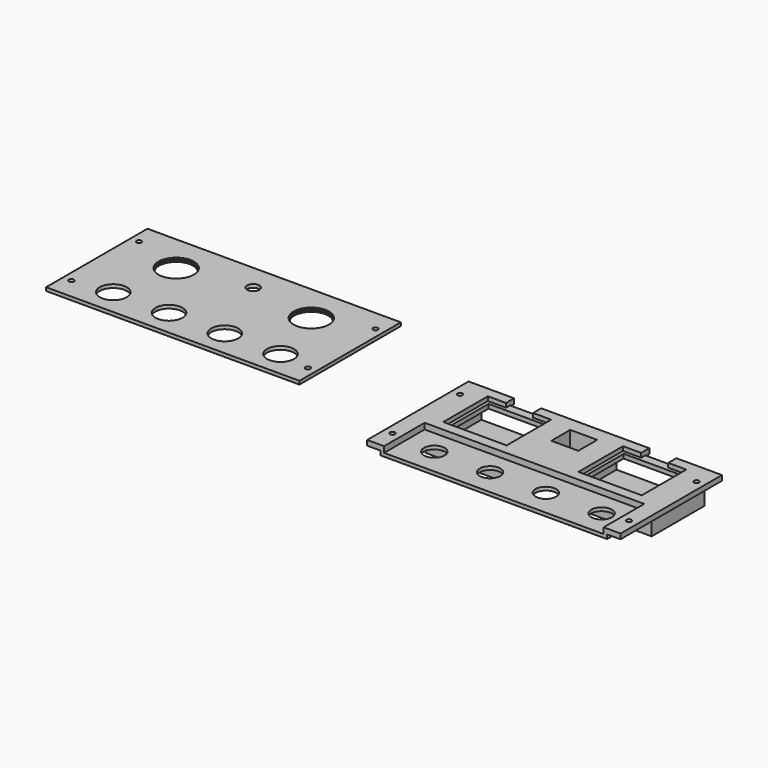
from build123d import *

# Parameters (mm, degrees)
F0_W      = 150
F0_H      = 75
F0_R      = 1.5
F0_R_2    = 6.1
F0_W_2    = 33.5
F0_H_2    = 29
F0_W_3    = 16
F0_H_3    = 8
F1_DEPTH  = 2
F2_W      = 10
F2_H      = 75
F3_DEPTH  = 3.5
F4_W      = 8
F4_H      = 2.5
F5_DEPTH  = 80
F6_W      = 130
F6_H      = 45
F6_W_2    = 33.5
F6_H_2    = 29
F6_W_3    = 16
F6_H_3    = 14
F7_DEPTH  = 3.5
F8_W      = 33.5
F8_H      = 29
F8_W_2    = 16
F8_H_2    = 9
F8_H_3    = 6
F9_DEPTH  = 2.5
F10_W     = 150
F10_H     = 75
F10_R     = 1.5
F10_R_2   = 8
F10_R_3   = 10
F10_R_4   = 3.6
F11_DEPTH = 2
F12_R     = 10.5
F13_DEPTH = 1
F14_W     = 26
F14_H     = 25
F15_DEPTH = 4.5
F16_W     = 16
F16_H     = 14
F17_DEPTH = 9
F18_W     = 134
F18_H     = 3
F19_DEPTH = 2.5
F20_W     = 54
F20_H     = 39
F20_W_2   = 33.5
F20_H_2   = 29
F21_DEPTH = 12
F22_W     = 50
F22_H     = 10.5
F23_DEPTH = 37
F24_R     = 1.5
F25_DEPTH = 25
F26_W     = 16
F26_H     = 3
F27_DEPTH = 3


# Not quite as in the source:
# - a feature names something its author has since deleted; it is built from what else it names


with BuildPart() as f1:
    # F0 (on Top) → F1 (new body)
    with BuildSketch(Plane.XY):
        Rectangle(F0_W, F0_H)
        with Locations((-70, -25)):
            Circle(F0_R, mode=Mode.SUBTRACT)
        with Locations((-47.6297214627, -22)):
            Circle(F0_R_2, mode=Mode.SUBTRACT)
        with Locations((-14.6297214627, -22)):
            Circle(F0_R_2, mode=Mode.SUBTRACT)
        with Locations((18.3702785373, -22)):
            Circle(F0_R_2, mode=Mode.SUBTRACT)
        with Locations((51.3702785373, -22)):
            Circle(F0_R_2, mode=Mode.SUBTRACT)
        with Locations((70, -25)):
            Circle(F0_R, mode=Mode.SUBTRACT)
        with Locations((-40, 15)):
            Rectangle(F0_W_2, F0_H_2, mode=Mode.SUBTRACT)
        with Locations((-70, 25)):
            Circle(F0_R, mode=Mode.SUBTRACT)
        with Locations((40, 15)):
            Rectangle(F0_W_2, F0_H_2, mode=Mode.SUBTRACT)
        Polygon((8, 18), (8, 15), (-8, 15), (-8, 18), (-8, 26), (-8, 29), (8, 29), (8, 26), align=None, mode=Mode.SUBTRACT)
        with Locations((70, 25)):
            Circle(F0_R, mode=Mode.SUBTRACT)
        with Locations((0, 22)):
            Rectangle(F0_W_3, F0_H_3)
    extrude(amount=F1_DEPTH)

    # F2 (on face) → F3 (join)
    with BuildSketch(Plane.XY.offset(2)):
        with Locations((-70, 0)):
            Rectangle(F2_W, F2_H)
        with Locations((70, 0)):
            Rectangle(F2_W, F2_H)
    extrude(amount=F3_DEPTH)

    # F4 (on face) → F5 (cut)
    with BuildSketch(Plane.XZ.offset(37.5)):
        with Locations((-71, 1.25)):
            Rectangle(F4_W, F4_H)
        with Locations((71, 1.25)):
            Rectangle(F4_W, F4_H)
    extrude(amount=-F5_DEPTH, mode=Mode.SUBTRACT)

    # F6 (on face) → F7 (join)
    with BuildSketch(Plane.XY.offset(2)):
        with Locations((0, 15)):
            Rectangle(F6_W, F6_H)
        with Locations((-40, 15)):
            Rectangle(F6_W_2, F6_H_2, mode=Mode.SUBTRACT)
        with Locations((0, 22)):
            Rectangle(F6_W_3, F6_H_3, mode=Mode.SUBTRACT)
        with Locations((40, 15)):
            Rectangle(F6_W_2, F6_H_2, mode=Mode.SUBTRACT)
    extrude(amount=F7_DEPTH)

    # F8 (on face) → F9 (cut)
    with BuildSketch(Plane.XY.offset(5.5)):
        Polygon((-58.75, -1.5), (-21.25, -1.5), (-21.25, 31.5), (-32, 31.5), (-48, 31.5), (-58.75, 31.5), align=None)
        with Locations((-40, 15)):
            Rectangle(F8_W, F8_H, mode=Mode.SUBTRACT)
        Polygon((48, 31.5), (32, 31.5), (21.25, 31.5), (21.25, -1.5), (58.75, -1.5), (58.75, 31.5), align=None)
        with Locations((40, 15)):
            Rectangle(F8_W, F8_H, mode=Mode.SUBTRACT)
        with Locations((-40, 42)):
            Rectangle(F8_W_2, F8_H_2)
        with Locations((40, 42)):
            Rectangle(F8_W_2, F8_H_2)
        with Locations((-40, 34.5)):
            Rectangle(F8_W_2, F8_H_3)
        with Locations((40, 34.5)):
            Rectangle(F8_W_2, F8_H_3)
    extrude(amount=-F9_DEPTH, mode=Mode.SUBTRACT)

    # F14 (on face) + F0 (on Top) → F15 (join)
    with BuildSketch(Plane.XY):
        with Locations((0, 22)):
            Rectangle(F14_W, F14_H)
        Polygon((8, 29), (8, 26), (8, 18), (8, 15), (-8, 15), (-8, 18), (-8, 26), (-8, 29), align=None, mode=Mode.SUBTRACT)
    with BuildSketch(Plane.XY):
        with Locations((0, 22)):
            Rectangle(F0_W_3, F0_H_3)
    extrude(amount=-F15_DEPTH)

    # F16 (on face) → F17 (cut)
    with BuildSketch(Plane.XY.offset(5.5)):
        with Locations((0, 22)):
            Rectangle(F16_W, F16_H)
    extrude(amount=-F17_DEPTH, mode=Mode.SUBTRACT)

    # F18 (on face) → F19 (cut)
    with BuildSketch(Plane.XY):
        with Locations((0, 36)):
            Rectangle(F18_W, F18_H)
    extrude(amount=F19_DEPTH, mode=Mode.SUBTRACT)

    # F20 (on face) → F21 (join)
    with BuildSketch(Plane.XY):
        with Locations((40, 15)):
            Rectangle(F20_W, F20_H)
        with Locations((40, 15)):
            Rectangle(F20_W_2, F20_H_2, mode=Mode.SUBTRACT)
        with Locations((-40, 15)):
            Rectangle(F20_W, F20_H)
        with Locations((-40, 15)):
            Rectangle(F20_W_2, F20_H_2, mode=Mode.SUBTRACT)
        with Locations((40, 15)):
            Rectangle(F20_W_2, F20_H_2)
        with Locations((-40, 15)):
            Rectangle(F20_W_2, F20_H_2)
    extrude(amount=-F21_DEPTH)

    # F22 (on face) → F23 (cut)
    with BuildSketch(Plane(origin=(0, 34.5, 0), x_dir=(-1, 0, 0), z_dir=(0, 1, 0))):
        with Locations((-40, -4.75)):
            Rectangle(F22_W, F22_H)
        with Locations((40, -4.75)):
            Rectangle(F22_W, F22_H)
    extrude(amount=-F23_DEPTH, mode=Mode.SUBTRACT)

    # F24 (on face) → F25 (cut)
    with BuildSketch(Plane.XY.offset(5.5)):
        with Locations((-70, 25)):
            Circle(F24_R)
        with Locations((-70, -25)):
            Circle(F24_R)
        with Locations((70, 25)):
            Circle(F24_R)
        with Locations((70, -25)):
            Circle(F24_R)
    extrude(amount=-F25_DEPTH, mode=Mode.SUBTRACT)

    # F26 (on face) → F27 (cut)
    with BuildSketch(Plane.XY.offset(3)):
        with Locations((-40, 36)):
            Rectangle(F26_W, F26_H)
        with Locations((40, 36)):
            Rectangle(F26_W, F26_H)
    extrude(amount=-F27_DEPTH, mode=Mode.SUBTRACT)


with BuildPart() as f11:
    # F10 (on Top) → F11 (new body)
    with BuildSketch(Plane.XY):
        with Locations((-215.6192851201, 31.9309936473)):
            Rectangle(F10_W, F10_H)
        with Locations((-285.6192851201, 6.9309936473)):
            Circle(F10_R, mode=Mode.SUBTRACT)
        with Locations((-263.2490065828, 9.9309936473)):
            Circle(F10_R_2, mode=Mode.SUBTRACT)
        with Locations((-230.2490065828, 9.9309936473)):
            Circle(F10_R_2, mode=Mode.SUBTRACT)
        with Locations((-197.2490065828, 9.9309936473)):
            Circle(F10_R_2, mode=Mode.SUBTRACT)
        with Locations((-164.2490065828, 9.9309936473)):
            Circle(F10_R_2, mode=Mode.SUBTRACT)
        with Locations((-145.6192851201, 6.9309936473)):
            Circle(F10_R, mode=Mode.SUBTRACT)
        with Locations((-255.6192851201, 46.9309936473)):
            Circle(F10_R_3, mode=Mode.SUBTRACT)
        with Locations((-285.6192851201, 56.9309936473)):
            Circle(F10_R, mode=Mode.SUBTRACT)
        with Locations((-175.6192851201, 46.9309936473)):
            Circle(F10_R_3, mode=Mode.SUBTRACT)
        with Locations((-215.6192851201, 53.9309936473)):
            Circle(F10_R_4, mode=Mode.SUBTRACT)
        with Locations((-145.6192851201, 56.9309936473)):
            Circle(F10_R, mode=Mode.SUBTRACT)
    extrude(amount=F11_DEPTH)

    # F12 (on face) → F13 (cut)
    with BuildSketch(Plane.XY.offset(2)):
        with Locations((-255.6192851201, 46.9309936473)):
            Circle(F12_R)
        with Locations((-175.6192851201, 46.9309936473)):
            Circle(F12_R)
    extrude(amount=-F13_DEPTH, mode=Mode.SUBTRACT)


solid = Compound([f1.part, f11.part])
